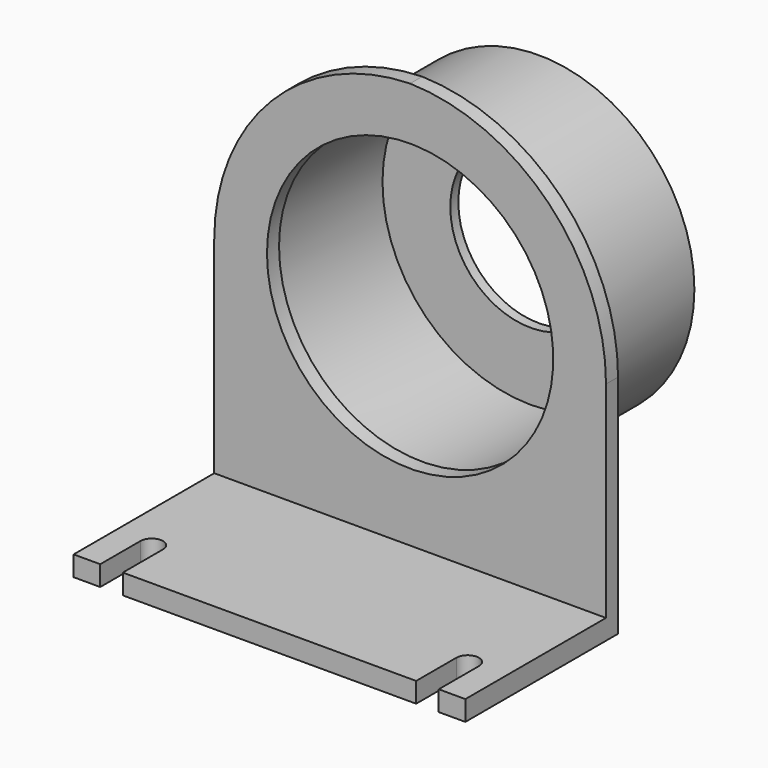
from build123d import *

# Parameters (mm, degrees)
F0_W        = 78
F0_H        = 38
F1_DEPTH    = 4
F2_W        = 78
F2_H        = 3
F3_DEPTH    = 81
F4_T1_DEPTH = 203
F5_R        = 31
F5_R_2      = 29.5
F6_DEPTH    = 27
F7_R        = 28.5
F8_DEPTH    = 3
F9_R        = 31
F10_DEPTH   = 2
F11_R       = 16
F12_DEPTH   = 2
F14_DEPTH   = 4


# Not quite as in the source:
# - a fillet or chamfer that OpenCascade refuses, or shapes differently, is made with other operations: its cross-section is extruded or revolved along the edge and cut away or added


with BuildPart() as f1:
    # F0 (on Top) → F1 (new body)
    with BuildSketch(Plane.XY):
        Rectangle(F0_W, F0_H)
    extrude(amount=F1_DEPTH)

    # F2 (on face) → F3 (join)
    with BuildSketch(Plane.XY.offset(4)):
        with Locations((0, 17.5)):
            Rectangle(F2_W, F2_H)
    extrude(amount=F3_DEPTH)

    # F4: fillet of radius 40 on 2 edges, made by hand

    # F4_s2 → F4_t1 (cut)
    with BuildSketch(Plane.XZ.offset(-119)):
        with BuildLine():
            ThreePointArc((39, 45), (27.2842712475, 73.2842712475), (-1, 85))
            Line((-1, 85), (39, 85))
            Line((39, 85), (39, 45))
        make_face()
        with BuildLine():
            ThreePointArc((-39, 45), (-27.2842712475, 73.2842712475), (1, 85))
            Line((1, 85), (-39, 85))
            Line((-39, 85), (-39, 45))
        make_face()
    extrude(amount=F4_T1_DEPTH, mode=Mode.SUBTRACT)

    # F5 (on face) → F6 (join)
    with BuildSketch(Plane(origin=(0, 19, 0), x_dir=(-1, 0, 0), z_dir=(0, 1, 0))):
        with Locations((0, 45.9753048304)):
            Circle(F5_R)
        with Locations((0, 45.9753048304)):
            Circle(F5_R_2, mode=Mode.SUBTRACT)
    extrude(amount=F6_DEPTH)

    # F7 (on face) → F8 (cut, through all)
    with BuildSketch(Plane(origin=(0, 19, 0), x_dir=(-1, 0, 0), z_dir=(0, 1, 0))):
        with Locations((0, 45.9753048304)):
            Circle(F7_R)
    extrude(amount=-F8_DEPTH, mode=Mode.SUBTRACT)

    # F9 (on face) → F10 (join)
    with BuildSketch(Plane(origin=(0, 46, 0), x_dir=(-1, 0, 0), z_dir=(0, 1, 0))):
        with Locations((0, 45.9753048304)):
            Circle(F9_R)
    extrude(amount=F10_DEPTH)

    # F11 (on face) → F12 (cut, through all)
    with BuildSketch(Plane(origin=(0, 48, 0), x_dir=(-1, 0, 0), z_dir=(0, 1, 0))):
        with Locations((0, 45.9753048304)):
            Circle(F11_R)
    extrude(amount=-F12_DEPTH, mode=Mode.SUBTRACT)

    # F13 (on face) → F14 (cut, through all)
    with BuildSketch(Plane.XY.offset(4)):
        with BuildLine():
            Line((29.2, -19), (33.7, -19))
            Line((33.7, -19), (33.7, -9))
            ThreePointArc((33.7, -9), (31.45, -11.25), (29.2, -9))
            Line((29.2, -9), (29.2, -19))
        make_face()
        with BuildLine():
            ThreePointArc((29.2, -9), (31.45, -11.25), (33.7, -9))
            Line((33.7, -9), (29.2, -9))
        make_face()
        with BuildLine():
            Line((29.2, -9), (33.7, -9))
            ThreePointArc((33.7, -9), (31.45, -6.75), (29.2, -9))
        make_face()
        with BuildLine():
            ThreePointArc((-29.2, -9), (-31.45, -6.75), (-33.7, -9))
            Line((-33.7, -9), (-29.2, -9))
        make_face()
        with BuildLine():
            ThreePointArc((-29.2, -9), (-31.45, -11.25), (-33.7, -9))
            Line((-33.7, -9), (-33.7, -19))
            Line((-33.7, -19), (-29.2, -19))
            Line((-29.2, -19), (-29.2, -9))
        make_face()
        with BuildLine():
            Line((-29.2, -9), (-33.7, -9))
            ThreePointArc((-33.7, -9), (-31.45, -11.25), (-29.2, -9))
        make_face()
    extrude(amount=-F14_DEPTH, mode=Mode.SUBTRACT)


solid = f1.part
